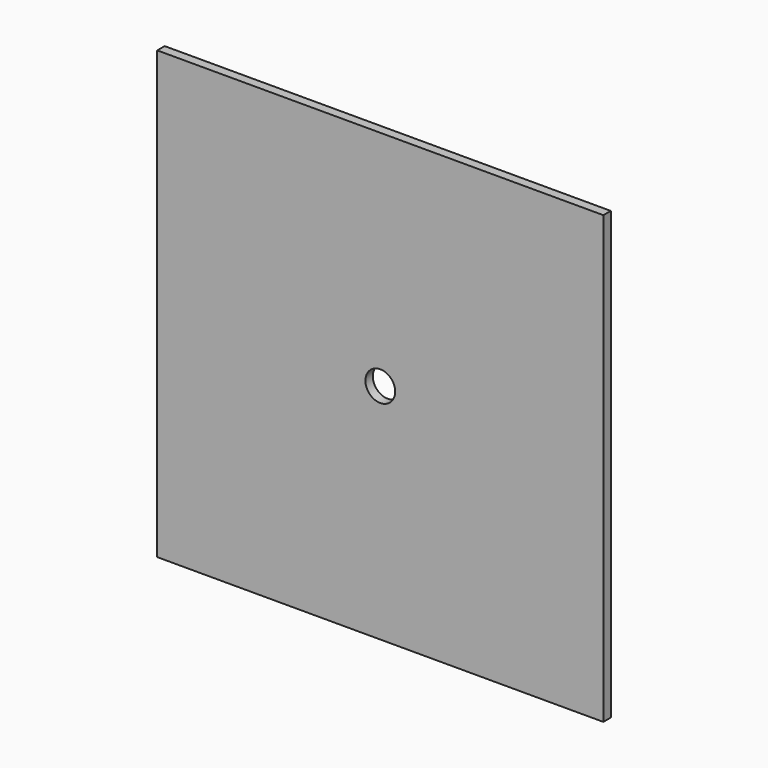
from build123d import *

# Parameters (mm, degrees)
F0_W     = 76.2
F0_H     = 76.2
F1_DEPTH = 1.5875
F2_R     = 2.54
F3_DEPTH = 25.4


# Not quite as in the source:
# - a length typed as a fraction of an inch, garbled in the dataset ("3 / 203.2 mm" for 3/8 in), is restored


with BuildPart() as f1:
    # F0 (on Front) → F1 (new body)
    with BuildSketch(Plane.XZ):
        Rectangle(F0_W, F0_H)
    extrude(amount=F1_DEPTH)

    # F2 (on face) → F3 (cut)
    with BuildSketch(Plane.XZ.offset(1.5875)):
        Circle(F2_R)
    extrude(amount=-F3_DEPTH, mode=Mode.SUBTRACT)


solid = f1.part
